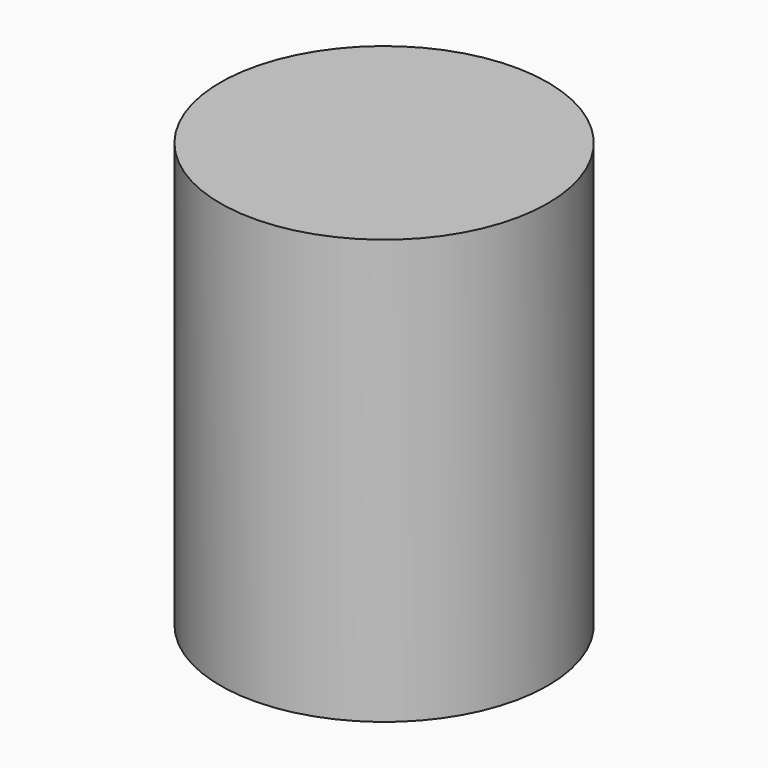
from build123d import *

# Parameters (mm, degrees)
F0_R     = 13.5
F1_DEPTH = 35
F2_R     = 13.05
F3_DEPTH = 3


# Not quite as in the source:
# - a feature names something its author has since deleted; it is built from what else it names


with BuildPart() as f1:
    # F0 (on Top) → F1 (new body)
    with BuildSketch(Plane.XY):
        Circle(F0_R)
    extrude(amount=F1_DEPTH)

    # F2 (on Top) → F3 (join)
    with BuildSketch(Plane.XY):
        Circle(F2_R)
    extrude(amount=F3_DEPTH)


solid = f1.part
